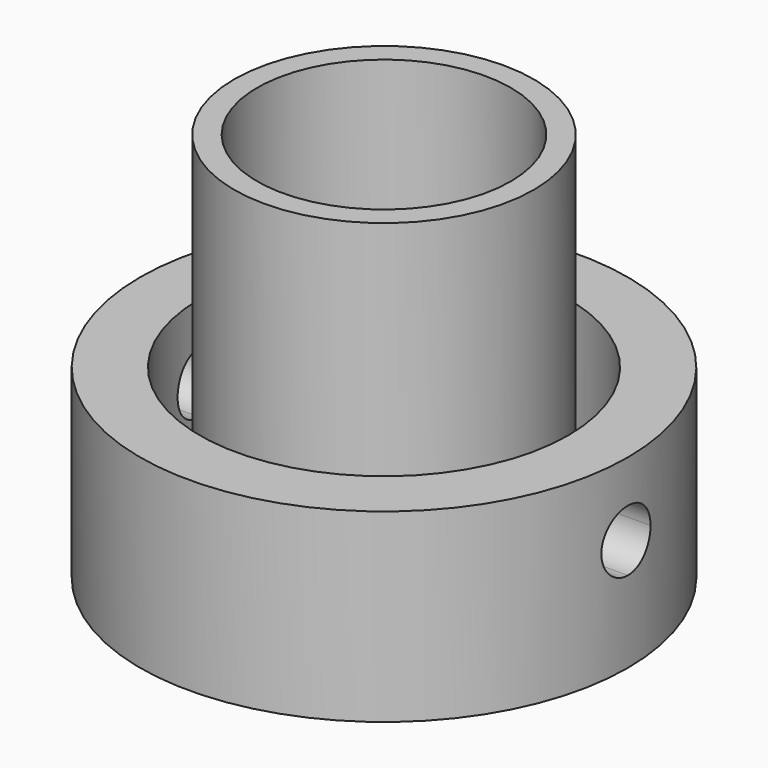
from build123d import *

# Parameters (mm, degrees)
F0_R          = 9.75
F1_DEPTH      = 25.4
F2_R          = 8.255
F3_DEPTH      = 25.4
F4_R          = 15.875
F4_R_2        = 9.75
F5_DEPTH      = 2.54
F6_R          = 15.875
F6_R_2        = 12
F7_DEPTH      = 9.525
F9_DEPTH      = 25.4
F9_DEPTH_BACK = 25.4


with BuildPart() as f1:
    # F0 (on Top) → F1 (new body)
    with BuildSketch(Plane.XY):
        Circle(F0_R)
    extrude(amount=F1_DEPTH)

    # F2 (on face) → F3 (cut)
    with BuildSketch(Plane.XY.offset(25.4)):
        Circle(F2_R)
    extrude(amount=-F3_DEPTH, mode=Mode.SUBTRACT)

    # F4 (on face) → F5 (join)
    with BuildSketch(Plane(origin=(0, 0, 0), x_dir=(1, 0, 0), z_dir=(0, 0, -1))):
        Circle(F4_R)
        Circle(F4_R_2, mode=Mode.SUBTRACT)
    extrude(amount=-F5_DEPTH)

    # F6 (on face) → F7 (join)
    with BuildSketch(Plane.XY.offset(2.54)):
        Circle(F6_R)
        Circle(F6_R_2, mode=Mode.SUBTRACT)
    extrude(amount=F7_DEPTH)

    # F8 (on Right) → F9 (cut, two sides)
    with BuildSketch(Plane.YZ) as f9_sk:
        with BuildLine():
            ThreePointArc((0, 5.3025), (1.4142135624, 5.8882864376), (2, 7.3025))
            ThreePointArc((2, 7.3025), (-1.4142135624, 8.7167135624), (0, 5.3025))
        make_face()
    extrude(amount=-F9_DEPTH, mode=Mode.SUBTRACT)
    extrude(f9_sk.sketch, amount=F9_DEPTH_BACK, mode=Mode.SUBTRACT)


solid = f1.part
